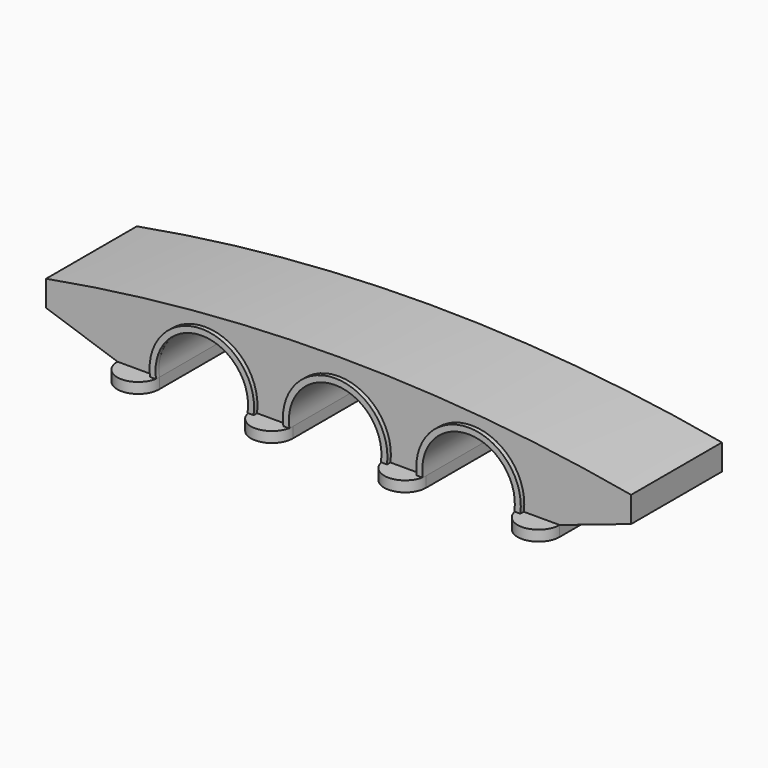
from build123d import *

# Parameters (mm, degrees)
F1_DEPTH = 65.69
F2_W     = 48.438
F2_H     = 131.38
F3_DEPTH = 12.26
F5_DEPTH = 5


# Not quite as in the source:
# - a feature names something its author has since deleted; it is built from what else it names


with BuildPart() as f1:
    # F0 (on Front) → F1 (new body, symmetric)
    with BuildSketch(Plane.XZ):
        with BuildLine():
            Line((-320.0353384018, 0), (-237.2032226722, -27.8760867547))
            Line((-237.2032226722, -27.8760867547), (-188.7652226722, -27.8760867547))
            ThreePointArc((-188.7652226722, -27.8760867547), (-135.7652226722, 33.6790422812), (-82.7652226722, -27.8760867547))
            Line((-82.7652226722, -27.8760867547), (-34.3272226722, -27.8760867547))
            ThreePointArc((-34.3272226722, -27.8760867547), (18.6727773278, 33.6324801702), (71.6727773278, -27.8760867547))
            Line((71.6727773278, -27.8760867547), (120.1107773278, -27.8760867547))
            ThreePointArc((120.1107773278, -27.8760867547), (173.1107773278, 33.6925448374), (226.1107773278, -27.8760867547))
            Line((226.1107773278, -27.8760867547), (274.5487773278, -27.8760867547))
            Line((274.5487773278, -27.8760867547), (357.3808930574, 0))
            Line((357.3808930574, 0), (357.3808930574, 29.795))
            ThreePointArc((357.3808930574, 29.795), (18.6727773278, 60.3473106454), (-320.0353384018, 29.795))
            Line((-320.0353384018, 29.795), (-320.0353384018, 0))
        make_face()
    extrude(amount=F1_DEPTH, both=True)

    # F2 (on face) → F3 (join)
    with BuildSketch(Plane(origin=(0, 0, -27.8760867547), x_dir=(1, 0, 0), z_dir=(0, 0, -1))):
        with BuildLine():
            ThreePointArc((-237.2286491756, -65.5376471925), (-213.0855863574, -89.7567669916), (-188.7906491756, -65.69))
            Line((-188.7906491756, -65.69), (-188.7906491756, 65.8423528075))
            ThreePointArc((-188.7906491756, 65.8423528075), (-212.8485010036, 90.3820549045), (-237.2286491756, 66.1625258279))
            Line((-237.2286491756, 66.1625258279), (-237.2286491756, -65.5376471925))
        make_face()
        with Locations((-58.5462226722, 0)):
            Rectangle(F2_W, F2_H)
        with BuildLine():
            Line((71.6727773278, 65.8423528075), (71.6727773278, -65.69))
            ThreePointArc((71.6727773278, -65.69), (95.8917773278, -89.909), (120.1107773278, -65.69))
            Line((120.1107773278, -65.69), (120.1107773278, 65.8423528075))
            ThreePointArc((120.1107773278, 65.8423528075), (95.8917773278, 90.0613528075), (71.6727773278, 65.8423528075))
        make_face()
        with BuildLine():
            Line((226.1107773278, 65.8423528075), (226.1107773278, -65.69))
            ThreePointArc((226.1107773278, -65.69), (250.3297773278, -89.909), (274.5487773278, -65.69))
            Line((274.5487773278, -65.69), (274.5487773278, 65.8423528075))
            ThreePointArc((274.5487773278, 65.8423528075), (250.3297773278, 90.0613528075), (226.1107773278, 65.8423528075))
        make_face()
        with BuildLine():
            Line((-34.3272226722, -65.69), (-82.7652226722, -65.69))
            ThreePointArc((-82.7652226722, -65.69), (-58.5462226722, -89.909), (-34.3272226722, -65.69))
        make_face()
        with BuildLine():
            ThreePointArc((-34.3272226722, 65.69), (-58.5462226722, 89.909), (-82.7652226722, 65.69))
            Line((-82.7652226722, 65.69), (-34.3272226722, 65.69))
        make_face()
    extrude(amount=F3_DEPTH)

    # F4 (on face) → F5 (join)
    with BuildSketch(Plane.XZ.offset(65.69)):
        with BuildLine():
            ThreePointArc((78.6827773278, -27.8760867547), (18.6727773278, 40.5462292936), (-41.3372226722, -27.8760867547))
            Line((-41.3372226722, -27.8760867547), (-34.3272226722, -27.8760867547))
            ThreePointArc((-34.3272226722, -27.8760867547), (18.6727773278, 33.6324801702), (71.6727773278, -27.8760867547))
            Line((71.6727773278, -27.8760867547), (78.6827773278, -27.8760867547))
        make_face()
        with BuildLine():
            ThreePointArc((233.1207773278, -27.8760867547), (173.1107773278, 40.5405201313), (113.1007773278, -27.8760867547))
            Line((113.1007773278, -27.8760867547), (120.1107773278, -27.8760867547))
            ThreePointArc((120.1107773278, -27.8760867547), (173.1107773278, 33.6925448374), (226.1107773278, -27.8760867547))
            Line((226.1107773278, -27.8760867547), (233.1207773278, -27.8760867547))
        make_face()
        with BuildLine():
            ThreePointArc((-188.7652226722, -27.8760867547), (-135.7652226722, 33.7954088447), (-82.7652226722, -27.8760867547))
            Line((-82.7652226722, -27.8760867547), (-75.7552226722, -27.8760867547))
            ThreePointArc((-75.7552226722, -27.8760867547), (-135.7652226722, 40.6185747484), (-195.7752226722, -27.8760867547))
            Line((-195.7752226722, -27.8760867547), (-188.7906491756, -27.8760867547))
            Line((-188.7906491756, -27.8760867547), (-188.7652226722, -27.8760867547))
        make_face()
    extrude(amount=F5_DEPTH)

    # F6: F1 across plane


with BuildPart() as f1_1:
    add(f1.part)
    add(f1.part.mirror(Plane.XZ))


solid = f1_1.part
